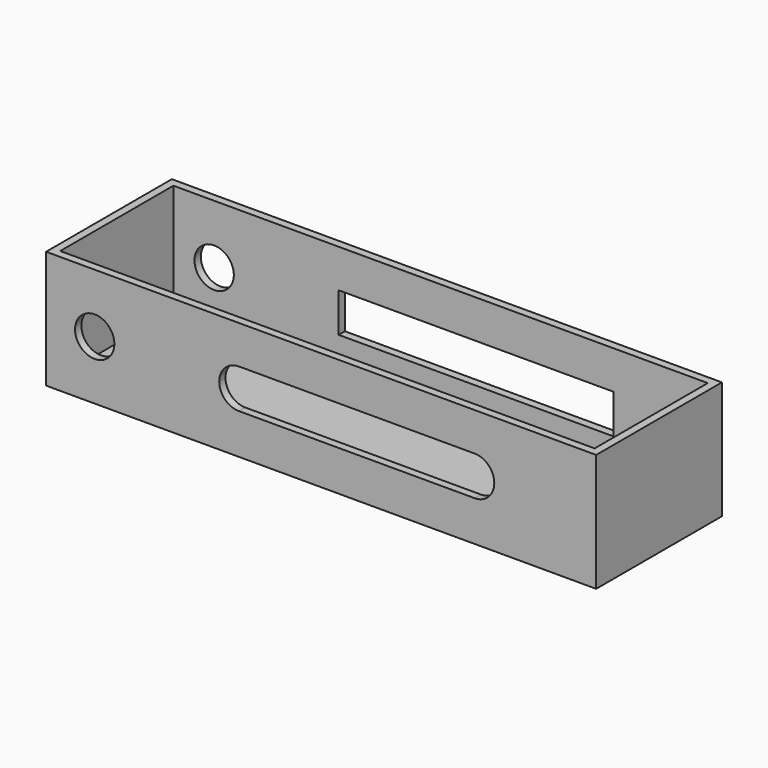
from build123d import *

# Parameters (mm, degrees)
F0_W     = 70
F0_H     = 20
F1_DEPTH = 15
F3_T     = -1
F4_D     = 5
F2_W     = 35
F2_H     = 5
F5_DEPTH = 25
F6_R     = 2.49999


# Not quite as in the source:
# - a fillet or chamfer is up to 0.001 mm smaller than in the source, because OpenCascade refuses the exact size


with BuildPart() as f1:
    # F0 (on Top) → F1 (new body)
    with BuildSketch(Plane.XY):
        with Locations((0, 1.5861968277)):
            Rectangle(F0_W, F0_H)
    extrude(amount=F1_DEPTH)

    # F3
    f3_openings = [f1.faces().sort_by_distance(p)[0] for p in [
        (0, 1.586197, 15),
    ]]
    offset(amount=F3_T, openings=f3_openings)

    # F4 (through all)
    with Locations(Plane.XZ.offset(8.4138031723)):
        with Locations((-28.8131628186, 7.5)):
            Hole(F4_D / 2)

    # F2 (on face) → F5 (cut)
    with BuildSketch(Plane.XZ.offset(8.4138031723)):
        with Locations((4.5323091745, 7.627816461)):
            Rectangle(F2_W, F2_H)
    extrude(amount=-F5_DEPTH, mode=Mode.SUBTRACT)

    # F6 (radius 2.5 in the source; OpenCascade refuses exactly that, so slightly less here)
    f6_edges = [f1.edges().sort_by_distance(p)[0] for p in [
        (-12.967691, -7.913803, 10.127816),
        (-12.967691, -7.913803, 5.127816),
        (22.032309, -7.913803, 5.127816),
        (22.032309, -7.913803, 10.127816),
    ]]
    fillet(f6_edges, radius=F6_R)


solid = f1.part
